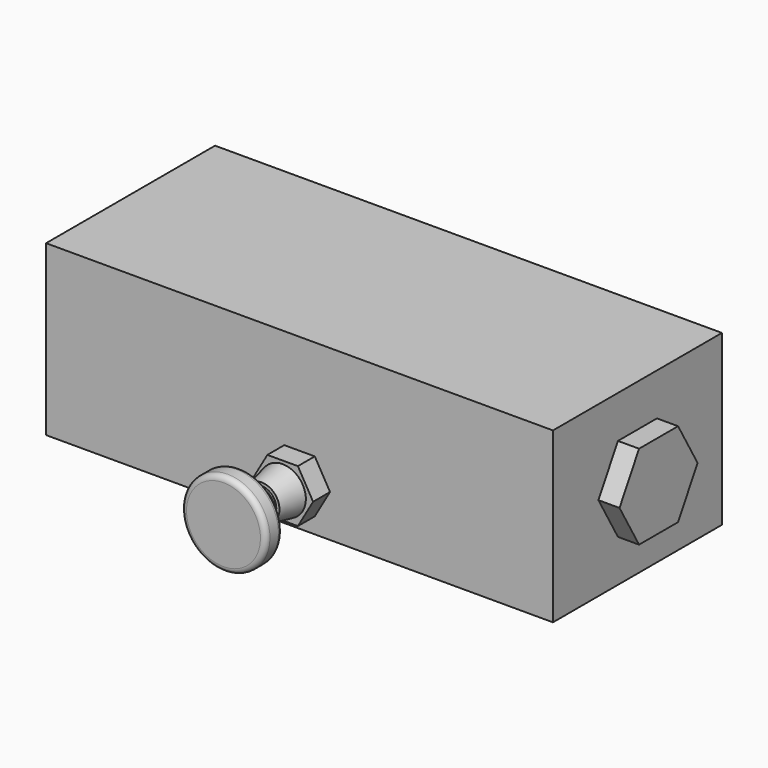
from build123d import *

# Parameters (mm, degrees)
F0_W          = 63.5
F0_H          = 50.8
F1_DEPTH      = 76.2
F1_DEPTH_BACK = 76.2
F3_DEPTH      = 6.35
F8_DEPTH      = 6.35


# Not quite as in the source:
# - a feature names something its author has since deleted; it is built from what else it names
# - the program builds the solid bodies; features that only make, move or delete a surface that nothing else refers to are left out


with BuildPart() as f1:
    # F0 (on Right) → F1 (new body, two sides)
    with BuildSketch(Plane.YZ) as f1_sk:
        Rectangle(F0_W, F0_H)
    extrude(amount=F1_DEPTH)
    extrude(f1_sk.sketch, amount=-F1_DEPTH_BACK)

    # F2 (on face) → F3 (join)
    with BuildSketch(Plane(origin=(-76.2, 0, 0), x_dir=(0, -1, 0), z_dir=(-1, 0, 0))):
        Polygon((7.3323484187, 12.7), (-7.3323484187, 12.7), (-14.6646968374, 0), (-7.3323484187, -12.7), (7.3323484187, -12.7), (14.6646968374, 0), align=None)
    extrude(amount=F3_DEPTH)


with BuildPart() as f6_1:
    # F6: instance of F1
    add(f1.part.mirror(Plane.YZ))


with BuildPart() as f8:
    # F7 (on face) → F8 (new body)
    with BuildSketch(Plane.XZ.offset(31.75)):
        Polygon((9.1654355234, -12.7), (4.5827177617, -4.7625), (-4.5827177617, -4.7625), (-9.1654355234, -12.7), (-4.5827177617, -20.6375), (4.5827177617, -20.6375), align=None)
    extrude(amount=F8_DEPTH)

    # F9 (on Right) → F10 (revolve)
    with BuildSketch(Plane.YZ):
        with BuildLine():
            Line((-38.1, -12.7), (-38.1, -5.715))
            Line((-38.1, -5.715), (-46.0375, -7.3025))
            Line((-46.0375, -7.3025), (-46.0375, -8.255))
            Line((-46.0375, -8.255), (-47.625, -8.255))
            Line((-47.625, -8.255), (-47.625, -7.3025))
            Line((-47.625, -7.3025), (-50.8, -7.3025))
            ThreePointArc((-50.8, -7.3025), (-53.0450640303, -6.3725640303), (-53.975, -4.1275))
            Line((-53.975, -4.1275), (-53.975, -1.5875))
            ThreePointArc((-53.975, -1.5875), (-54.4399679849, -0.4649679849), (-55.5625, 0))
            Line((-55.5625, 0), (-58.7375, 0))
            ThreePointArc((-58.7375, 0), (-59.8600320151, -0.4649679849), (-60.325, -1.5875))
            Line((-60.325, -1.5875), (-60.325, -12.7))
            Line((-60.325, -12.7), (-38.1, -12.7))
        make_face()
    revolve(axis=Axis((0, -65.4494816124, -12.7), (0, -1, 0)))


solid = Compound([f1.part, f6_1.part, f8.part])
